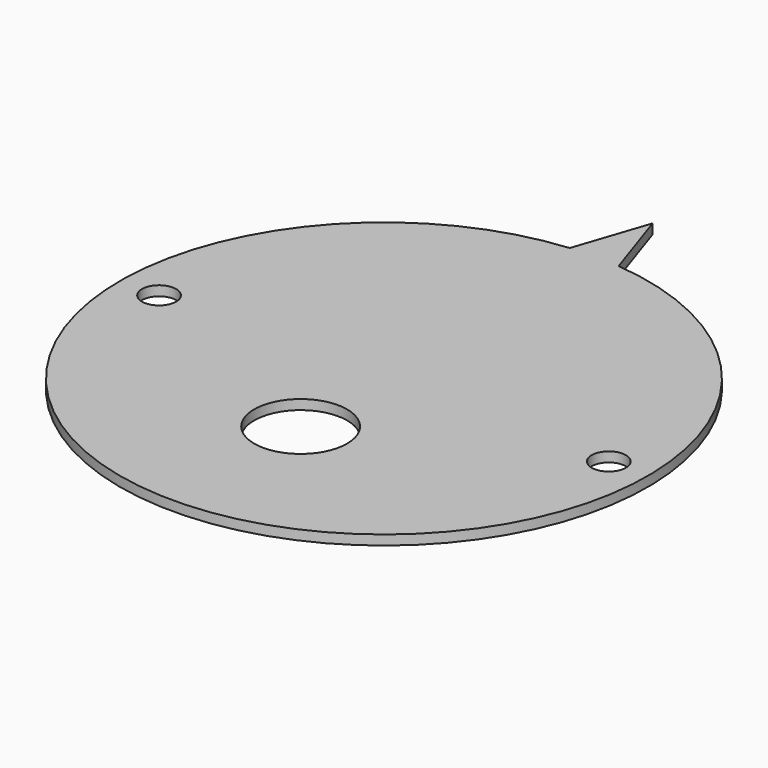
from build123d import *

# Parameters (mm, degrees)
F0_R       = 1.75
F0_R_2     = 4.75
F1_DEPTH   = 1
F2_SIZE2   = 2.5
F2_SIZE    = 7.465
F2_2_SIZE2 = 2.49999
F2_2_SIZE  = 7.46499


# Not quite as in the source:
# - a fillet or chamfer is up to 0.001 mm smaller than in the source, because OpenCascade refuses the exact size


with BuildPart() as f1:
    # F0 (on Top) → F1 (new body)
    with BuildSketch(Plane.XY):
        with BuildLine():
            Line((-2.5, 34.35), (-2.5, 26.8840101175))
            ThreePointArc((-2.5, 26.8840101175), (0, -27), (2.5, 26.8840101175))
            Line((2.5, 26.8840101175), (2.5, 34.35))
            Line((2.5, 34.35), (-2.5, 34.35))
        make_face()
        with Locations((-23, 0)):
            Circle(F0_R, mode=Mode.SUBTRACT)
        with Locations((0, -10.65)):
            Circle(F0_R_2, mode=Mode.SUBTRACT)
        with Locations((23, 0)):
            Circle(F0_R, mode=Mode.SUBTRACT)
    extrude(amount=F1_DEPTH)

    # F2
    f2_edges = [f1.edges().sort_by_distance(p)[0] for p in [
        (-2.5, 34.35, 0.5),
    ]]
    f2_side = f1.faces().sort_by_distance((-2.5, 30.617005, 0.5))[0]
    chamfer(f2_edges, length=F2_SIZE, length2=F2_SIZE2, reference=f2_side)

    # F2#2 (size 7.465 and 2.5 in the source; OpenCascade refuses exactly that, so slightly less here)
    f2_2_edges = [f1.edges().sort_by_distance(p)[0] for p in [
        (2.5, 34.35, 0.5),
    ]]
    f2_2_side = f1.faces().sort_by_distance((2.5, 30.617005, 0.5))[0]
    chamfer(f2_2_edges, length=F2_2_SIZE, length2=F2_2_SIZE2, reference=f2_2_side)


solid = f1.part
